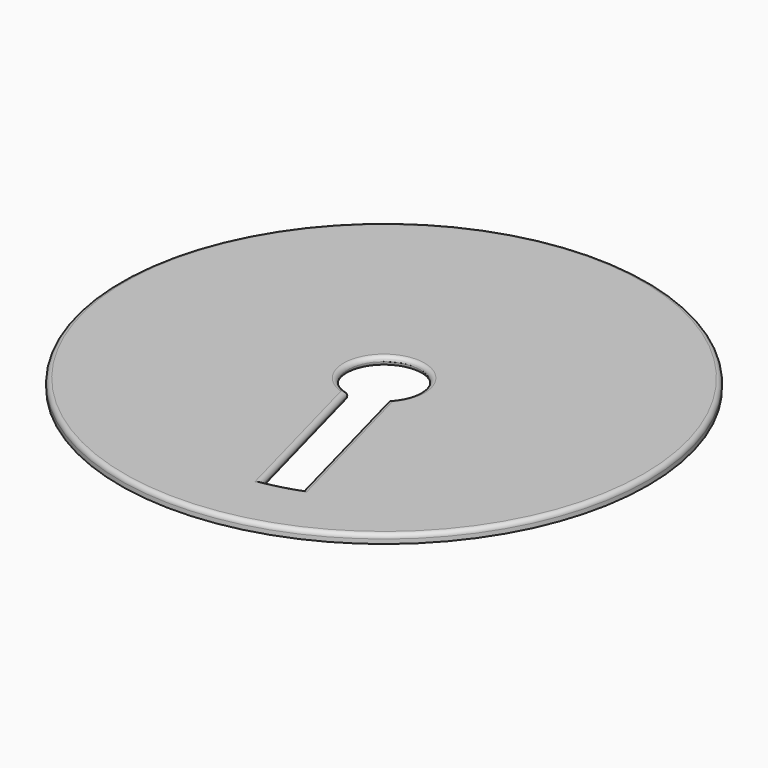
from build123d import *

# Parameters (mm, degrees)
F1_R     = 30
F1_R_2   = 29
F2_DEPTH = 1
F3_DEPTH = 1
F5_DEPTH = 1
F6_DEPTH = 0.7
F8_DEPTH = 1
F9_R     = 0.49999


# Not quite as in the source:
# - a fillet or chamfer is up to 0.001 mm smaller than in the source, because OpenCascade refuses the exact size
# - a feature names something its author has since deleted; it is built from what else it names


with BuildPart() as f2:
    # F1 (on Top) → F2 (new body)
    with BuildSketch(Plane.XY):
        Circle(F1_R)
        Circle(F1_R_2, mode=Mode.SUBTRACT)
    extrude(amount=F2_DEPTH)

    # F1 (on Top) → F3 (join)
    with BuildSketch(Plane.XY):
        Circle(F1_R)
        Circle(F1_R_2, mode=Mode.SUBTRACT)
        Circle(F1_R_2)
    extrude(amount=F3_DEPTH)

    # F4 (on Top) → F5 (join)
    with BuildSketch(Plane.XY):
        with BuildLine():
            ThreePointArc((-23.1384227377, 14.225), (-23.3296108799, 14.9578106993), (-23.8544380991, 15.5038151104))
            ThreePointArc((-23.8544380991, 15.5038151104), (-23.9897856273, 15.2935504561), (-24.123279831, 15.0821043027))
            ThreePointArc((-24.123279831, 15.0821043027), (-23.7680369305, 14.7173703349), (-23.6384227377, 14.225))
            ThreePointArc((-23.6384227377, 14.225), (-24.130831685, 13.3634018783), (-25.1231253841, 13.3503210049))
            ThreePointArc((-25.1231253841, 13.3503210049), (-25.2394960227, 13.1289885565), (-25.3539167907, 12.9066418316))
            ThreePointArc((-25.3539167907, 12.9066418316), (-23.8713637698, 12.9359613893), (-23.1384227377, 14.225))
        make_face()
        with BuildLine():
            ThreePointArc((-24.123279831, 15.0821043027), (-23.9897856273, 15.2935504561), (-23.8544380991, 15.5038151104))
            ThreePointArc((-23.8544380991, 15.5038151104), (-25.9374608433, 14.975), (-25.3539167907, 12.9066418316))
            ThreePointArc((-25.3539167907, 12.9066418316), (-25.2394960227, 13.1289885565), (-25.1231253841, 13.3503210049))
            ThreePointArc((-25.1231253841, 13.3503210049), (-25.5044481415, 14.725), (-24.123279831, 15.0821043027))
        make_face()
        with BuildLine():
            ThreePointArc((-1.4994786916, 28.410456942), (0, 26.95), (1.4994786916, 28.410456942))
            ThreePointArc((1.4994786916, 28.410456942), (1.2497103954, 28.4225390127), (0.9998455532, 28.4324253076))
            ThreePointArc((0.9998455532, 28.4324253076), (0, 27.45), (-0.9998455532, 28.4324253076))
            ThreePointArc((-0.9998455532, 28.4324253076), (-1.2497103954, 28.4225390127), (-1.4994786916, 28.410456942))
        make_face()
        with BuildLine():
            ThreePointArc((0.9998455532, 28.4324253076), (1.2497103954, 28.4225390127), (1.4994786916, 28.410456942))
            ThreePointArc((1.4994786916, 28.410456942), (1.4998696672, 28.4302267529), (1.5, 28.45))
            ThreePointArc((1.5, 28.45), (-0.0197732471, 29.9498696672), (-1.4994786916, 28.410456942))
            ThreePointArc((-1.4994786916, 28.410456942), (-1.2497103954, 28.4225390127), (-0.9998455532, 28.4324253076))
            ThreePointArc((-0.9998455532, 28.4324253076), (-0.0087876855, 29.4499613875), (1, 28.45))
            ThreePointArc((1, 28.45), (0.9999613875, 28.4412123145), (0.9998455532, 28.4324253076))
        make_face()
        with BuildLine():
            ThreePointArc((25.1231253841, 13.3503210049), (25.2394960227, 13.1289885565), (25.3539167907, 12.9066418316))
            ThreePointArc((25.3539167907, 12.9066418316), (25.9274613483, 13.4579410321), (26.1384227377, 14.225))
            ThreePointArc((26.1384227377, 14.225), (25.371233437, 15.5338118577), (23.8544380991, 15.5038151104))
            ThreePointArc((23.8544380991, 15.5038151104), (23.9897856273, 15.2935504561), (24.123279831, 15.0821043027))
            ThreePointArc((24.123279831, 15.0821043027), (25.1307930725, 15.0953858072), (25.6384227377, 14.225))
            ThreePointArc((25.6384227377, 14.225), (25.5000208593, 13.7174089473), (25.1231253841, 13.3503210049))
        make_face()
        with BuildLine():
            ThreePointArc((23.8544380991, 15.5038151104), (23.339384632, 13.475), (25.3539167907, 12.9066418316))
            ThreePointArc((25.3539167907, 12.9066418316), (25.2394960227, 13.1289885565), (25.1231253841, 13.3503210049))
            ThreePointArc((25.1231253841, 13.3503210049), (23.7723973339, 13.725), (24.123279831, 15.0821043027))
            ThreePointArc((24.123279831, 15.0821043027), (23.9897856273, 15.2935504561), (23.8544380991, 15.5038151104))
        make_face()
        with BuildLine():
            ThreePointArc((-24.123279831, -15.0821043027), (-23.9897856273, -15.2935504561), (-23.8544380991, -15.5038151104))
            ThreePointArc((-23.8544380991, -15.5038151104), (-23.3296108799, -14.9578106993), (-23.1384227377, -14.225))
            ThreePointArc((-23.1384227377, -14.225), (-23.8713637698, -12.9359613893), (-25.3539167907, -12.9066418316))
            ThreePointArc((-25.3539167907, -12.9066418316), (-25.2394960227, -13.1289885565), (-25.1231253841, -13.3503210049))
            ThreePointArc((-25.1231253841, -13.3503210049), (-24.130831685, -13.3634018783), (-23.6384227377, -14.225))
            ThreePointArc((-23.6384227377, -14.225), (-23.7680369305, -14.7173703349), (-24.123279831, -15.0821043027))
        make_face()
        with BuildLine():
            ThreePointArc((-25.3539167907, -12.9066418316), (-25.9374608433, -14.975), (-23.8544380991, -15.5038151104))
            ThreePointArc((-23.8544380991, -15.5038151104), (-23.9897856273, -15.2935504561), (-24.123279831, -15.0821043027))
            ThreePointArc((-24.123279831, -15.0821043027), (-25.5044481415, -14.725), (-25.1231253841, -13.3503210049))
            ThreePointArc((-25.1231253841, -13.3503210049), (-25.2394960227, -13.1289885565), (-25.3539167907, -12.9066418316))
        make_face()
        with BuildLine():
            ThreePointArc((1.0415869357, -28.4309267639), (1.2705740372, -28.4216139868), (1.4994786916, -28.410456942))
            ThreePointArc((1.4994786916, -28.410456942), (0, -26.95), (-1.4994786916, -28.410456942))
            ThreePointArc((-1.4994786916, -28.410456942), (-1.2705740372, -28.4216139868), (-1.0415869357, -28.4309267639))
            Line((-1.0415869357, -28.4309267639), (0, -27.3893398282))
            Line((0, -27.3893398282), (1.0415869357, -28.4309267639))
        make_face()
        with BuildLine():
            ThreePointArc((1.5, -28.45), (1.4998696672, -28.4302267529), (1.4994786916, -28.410456942))
            ThreePointArc((1.4994786916, -28.410456942), (1.2705740372, -28.4216139868), (1.0415869357, -28.4309267639))
            Line((1.0415869357, -28.4309267639), (1.0606601718, -28.45))
            Line((1.0606601718, -28.45), (0, -29.5106601718))
            Line((0, -29.5106601718), (-1.0606601718, -28.45))
            Line((-1.0606601718, -28.45), (-1.0415869357, -28.4309267639))
            ThreePointArc((-1.0415869357, -28.4309267639), (-1.2705740372, -28.4216139868), (-1.4994786916, -28.410456942))
            ThreePointArc((-1.4994786916, -28.410456942), (-0.0197732471, -29.9498696672), (1.5, -28.45))
        make_face()
        with BuildLine():
            ThreePointArc((26.1384227377, -14.225), (25.9274613483, -13.4579410321), (25.3539167907, -12.9066418316))
            ThreePointArc((25.3539167907, -12.9066418316), (25.2394960227, -13.1289885565), (25.1231253841, -13.3503210049))
            ThreePointArc((25.1231253841, -13.3503210049), (25.5000208593, -13.7174089473), (25.6384227377, -14.225))
            ThreePointArc((25.6384227377, -14.225), (25.1307930725, -15.0953858072), (24.123279831, -15.0821043027))
            ThreePointArc((24.123279831, -15.0821043027), (23.9897856273, -15.2935504561), (23.8544380991, -15.5038151104))
            ThreePointArc((23.8544380991, -15.5038151104), (25.371233437, -15.5338118577), (26.1384227377, -14.225))
        make_face()
        with BuildLine():
            ThreePointArc((25.1231253841, -13.3503210049), (25.2394960227, -13.1289885565), (25.3539167907, -12.9066418316))
            ThreePointArc((25.3539167907, -12.9066418316), (23.339384632, -13.475), (23.8544380991, -15.5038151104))
            ThreePointArc((23.8544380991, -15.5038151104), (23.9897856273, -15.2935504561), (24.123279831, -15.0821043027))
            ThreePointArc((24.123279831, -15.0821043027), (23.7723973339, -13.725), (25.1231253841, -13.3503210049))
        make_face()
        with BuildLine():
            ThreePointArc((-23.6384227377, 14.225), (-23.7680369305, 14.7173703349), (-24.123279831, 15.0821043027))
            ThreePointArc((-24.123279831, 15.0821043027), (-24.6384227377, 14.225), (-25.1231253841, 13.3503210049))
            ThreePointArc((-25.1231253841, 13.3503210049), (-24.130831685, 13.3634018783), (-23.6384227377, 14.225))
        make_face()
        with BuildLine():
            ThreePointArc((-25.1231253841, 13.3503210049), (-24.6384227377, 14.225), (-24.123279831, 15.0821043027))
            ThreePointArc((-24.123279831, 15.0821043027), (-25.5044481415, 14.725), (-25.1231253841, 13.3503210049))
        make_face()
        with BuildLine():
            ThreePointArc((-0.9998455532, 28.4324253076), (0, 28.45), (0.9998455532, 28.4324253076))
            ThreePointArc((0.9998455532, 28.4324253076), (0.9999613875, 28.4412123145), (1, 28.45))
            ThreePointArc((1, 28.45), (-0.0087876855, 29.4499613875), (-0.9998455532, 28.4324253076))
        make_face()
        with BuildLine():
            ThreePointArc((-0.9998455532, 28.4324253076), (0, 27.45), (0.9998455532, 28.4324253076))
            ThreePointArc((0.9998455532, 28.4324253076), (0, 28.45), (-0.9998455532, 28.4324253076))
        make_face()
        with BuildLine():
            ThreePointArc((24.123279831, 15.0821043027), (24.6384227377, 14.225), (25.1231253841, 13.3503210049))
            ThreePointArc((25.1231253841, 13.3503210049), (25.5000208593, 13.7174089473), (25.6384227377, 14.225))
            ThreePointArc((25.6384227377, 14.225), (25.1307930725, 15.0953858072), (24.123279831, 15.0821043027))
        make_face()
        with BuildLine():
            ThreePointArc((24.123279831, 15.0821043027), (23.7723973339, 13.725), (25.1231253841, 13.3503210049))
            ThreePointArc((25.1231253841, 13.3503210049), (24.6384227377, 14.225), (24.123279831, 15.0821043027))
        make_face()
        with BuildLine():
            ThreePointArc((25.6384227377, -14.225), (25.5000208593, -13.7174089473), (25.1231253841, -13.3503210049))
            ThreePointArc((25.1231253841, -13.3503210049), (24.6384227377, -14.225), (24.123279831, -15.0821043027))
            ThreePointArc((24.123279831, -15.0821043027), (25.1307930725, -15.0953858072), (25.6384227377, -14.225))
        make_face()
        with BuildLine():
            ThreePointArc((24.123279831, -15.0821043027), (24.6384227377, -14.225), (25.1231253841, -13.3503210049))
            ThreePointArc((25.1231253841, -13.3503210049), (23.7723973339, -13.725), (24.123279831, -15.0821043027))
        make_face()
        with BuildLine():
            Line((1.0606601718, -28.45), (1.0415869357, -28.4309267639))
            ThreePointArc((1.0415869357, -28.4309267639), (0, -28.45), (-1.0415869357, -28.4309267639))
            Line((-1.0415869357, -28.4309267639), (-1.0606601718, -28.45))
            Line((-1.0606601718, -28.45), (0, -29.5106601718))
            Line((0, -29.5106601718), (1.0606601718, -28.45))
        make_face()
        with BuildLine():
            ThreePointArc((-25.1231253841, -13.3503210049), (-25.5044481415, -14.725), (-24.123279831, -15.0821043027))
            ThreePointArc((-24.123279831, -15.0821043027), (-24.6384227377, -14.225), (-25.1231253841, -13.3503210049))
        make_face()
        with BuildLine():
            ThreePointArc((-25.1231253841, -13.3503210049), (-24.6384227377, -14.225), (-24.123279831, -15.0821043027))
            ThreePointArc((-24.123279831, -15.0821043027), (-23.7680369305, -14.7173703349), (-23.6384227377, -14.225))
            ThreePointArc((-23.6384227377, -14.225), (-24.130831685, -13.3634018783), (-25.1231253841, -13.3503210049))
        make_face()
        with BuildLine():
            ThreePointArc((-1.0415869357, -28.4309267639), (0, -28.45), (1.0415869357, -28.4309267639))
            Line((1.0415869357, -28.4309267639), (0, -27.3893398282))
            Line((0, -27.3893398282), (-1.0415869357, -28.4309267639))
        make_face()
    extrude(amount=F5_DEPTH)

    # F4 (on Top) → F6 (cut)
    with BuildSketch(Plane.XY):
        with BuildLine():
            ThreePointArc((-25.1231253841, 13.3503210049), (-24.6384227377, 14.225), (-24.123279831, 15.0821043027))
            ThreePointArc((-24.123279831, 15.0821043027), (-25.5044481415, 14.725), (-25.1231253841, 13.3503210049))
        make_face()
        with BuildLine():
            ThreePointArc((-23.6384227377, 14.225), (-23.7680369305, 14.7173703349), (-24.123279831, 15.0821043027))
            ThreePointArc((-24.123279831, 15.0821043027), (-24.6384227377, 14.225), (-25.1231253841, 13.3503210049))
            ThreePointArc((-25.1231253841, 13.3503210049), (-24.130831685, 13.3634018783), (-23.6384227377, 14.225))
        make_face()
        with BuildLine():
            ThreePointArc((-0.9998455532, 28.4324253076), (0, 28.45), (0.9998455532, 28.4324253076))
            ThreePointArc((0.9998455532, 28.4324253076), (0.9999613875, 28.4412123145), (1, 28.45))
            ThreePointArc((1, 28.45), (-0.0087876855, 29.4499613875), (-0.9998455532, 28.4324253076))
        make_face()
        with BuildLine():
            ThreePointArc((-0.9998455532, 28.4324253076), (0, 27.45), (0.9998455532, 28.4324253076))
            ThreePointArc((0.9998455532, 28.4324253076), (0, 28.45), (-0.9998455532, 28.4324253076))
        make_face()
        with BuildLine():
            ThreePointArc((24.123279831, 15.0821043027), (23.7723973339, 13.725), (25.1231253841, 13.3503210049))
            ThreePointArc((25.1231253841, 13.3503210049), (24.6384227377, 14.225), (24.123279831, 15.0821043027))
        make_face()
        with BuildLine():
            ThreePointArc((24.123279831, 15.0821043027), (24.6384227377, 14.225), (25.1231253841, 13.3503210049))
            ThreePointArc((25.1231253841, 13.3503210049), (25.5000208593, 13.7174089473), (25.6384227377, 14.225))
            ThreePointArc((25.6384227377, 14.225), (25.1307930725, 15.0953858072), (24.123279831, 15.0821043027))
        make_face()
        with BuildLine():
            ThreePointArc((24.123279831, -15.0821043027), (24.6384227377, -14.225), (25.1231253841, -13.3503210049))
            ThreePointArc((25.1231253841, -13.3503210049), (23.7723973339, -13.725), (24.123279831, -15.0821043027))
        make_face()
        with BuildLine():
            ThreePointArc((25.6384227377, -14.225), (25.5000208593, -13.7174089473), (25.1231253841, -13.3503210049))
            ThreePointArc((25.1231253841, -13.3503210049), (24.6384227377, -14.225), (24.123279831, -15.0821043027))
            ThreePointArc((24.123279831, -15.0821043027), (25.1307930725, -15.0953858072), (25.6384227377, -14.225))
        make_face()
        with BuildLine():
            Line((1.0606601718, -28.45), (1.0415869357, -28.4309267639))
            ThreePointArc((1.0415869357, -28.4309267639), (0, -28.45), (-1.0415869357, -28.4309267639))
            Line((-1.0415869357, -28.4309267639), (-1.0606601718, -28.45))
            Line((-1.0606601718, -28.45), (0, -29.5106601718))
            Line((0, -29.5106601718), (1.0606601718, -28.45))
        make_face()
        with BuildLine():
            ThreePointArc((-1.0415869357, -28.4309267639), (0, -28.45), (1.0415869357, -28.4309267639))
            Line((1.0415869357, -28.4309267639), (0, -27.3893398282))
            Line((0, -27.3893398282), (-1.0415869357, -28.4309267639))
        make_face()
        with BuildLine():
            ThreePointArc((-25.1231253841, -13.3503210049), (-25.5044481415, -14.725), (-24.123279831, -15.0821043027))
            ThreePointArc((-24.123279831, -15.0821043027), (-24.6384227377, -14.225), (-25.1231253841, -13.3503210049))
        make_face()
        with BuildLine():
            ThreePointArc((-25.1231253841, -13.3503210049), (-24.6384227377, -14.225), (-24.123279831, -15.0821043027))
            ThreePointArc((-24.123279831, -15.0821043027), (-23.7680369305, -14.7173703349), (-23.6384227377, -14.225))
            ThreePointArc((-23.6384227377, -14.225), (-24.130831685, -13.3634018783), (-25.1231253841, -13.3503210049))
        make_face()
    extrude(amount=F6_DEPTH, mode=Mode.SUBTRACT)

    # F7 (on Top) → F8 (cut)
    with BuildSketch(Plane.XY):
        with BuildLine():
            ThreePointArc((2.8581924585, -2.9395128627), (3.7768101011, -1.595526703), (4.1, 0))
            ThreePointArc((4.1, 0), (-2.5186708329, 3.23516572), (-1.0055108466, -3.9747890431))
            ThreePointArc((-1.0055108466, -3.9747890431), (0.0287518116, -4.0998991858), (1.0611580849, -3.9602958878))
            ThreePointArc((1.0611580849, -3.9602958878), (2.0250497936, -3.5649927536), (2.8581924585, -2.9395128627))
        make_face()
        with BuildLine():
            ThreePointArc((1.0611580849, -3.9602958878), (0.0287518116, -4.0998991858), (-1.0055108466, -3.9747890431))
            Line((-1.0055108466, -3.9747890431), (3.8685251002, -22.1649388348))
            ThreePointArc((3.8685251002, -22.1649388348), (4.8507795796, -21.9708884088), (5.8234285148, -21.7333310915))
            Line((5.8234285148, -21.7333310915), (1.0611580849, -3.9602958878))
        make_face()
        with BuildLine():
            Line((7.7322284054, -21.1296626544), (2.8581924585, -2.9395128627))
            ThreePointArc((2.8581924585, -2.9395128627), (2.0250497936, -3.5649927536), (1.0611580849, -3.9602958878))
            Line((1.0611580849, -3.9602958878), (5.8234285148, -21.7333310915))
            ThreePointArc((5.8234285148, -21.7333310915), (6.7845458603, -21.4527372955), (7.7322284054, -21.1296626544))
        make_face()
    extrude(amount=F8_DEPTH, mode=Mode.SUBTRACT)

    # F9 (radius 0.5 in the source; OpenCascade refuses exactly that, so slightly less here)
    f9_edges = [f2.edges().sort_by_distance(p)[0] for p in [
        (-30, 0, 1),
        (-1.061158, 3.960296, 1),
        (1.431507, -13.069864, 1),
        (5.29521, -12.034588, 1),
        (5.29521, -12.034588, 0),
        (-1.061158, 3.960296, 0),
        (1.431507, -13.069864, 0),
        (5.823429, -21.733331, 1),
    ]]
    fillet(f9_edges, radius=F9_R)


solid = f2.part
